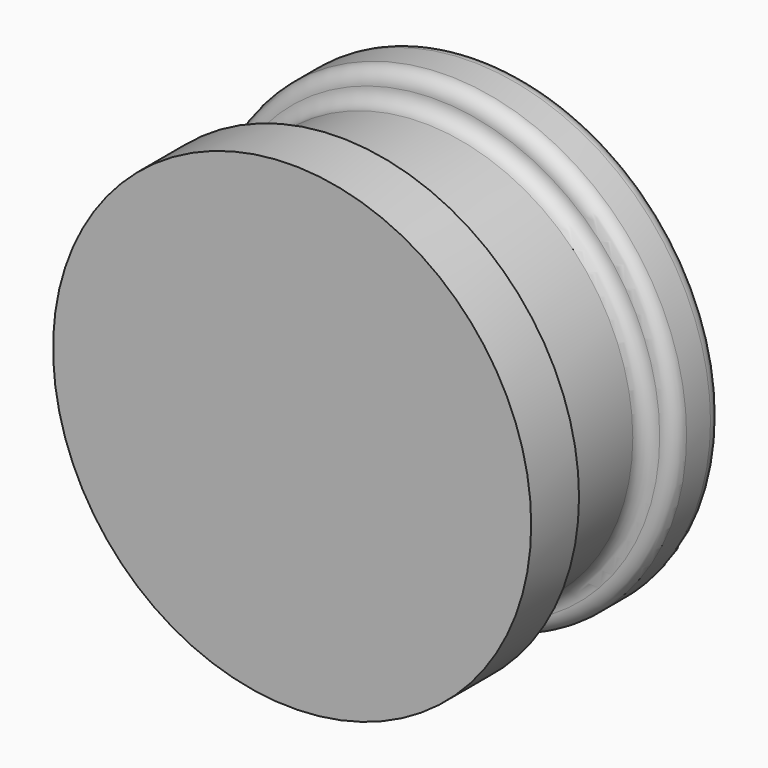
from build123d import *

# Parameters (mm, degrees)
F0_R      = 25.4
F1_DEPTH  = 6.35
F2_R      = 22.225
F3_DEPTH  = 12.7
F4_R      = 25.4
F4_R_2    = 22.225
F5_DEPTH  = 6.35
F7_D      = 3.175
F7_DEPTH  = 3.175
F7_TIP    = 0.9538662327
F8_D      = 12.7
F9_R      = 1.58749
F10_DEPTH = 6.35


# Not quite as in the source:
# - a fillet or chamfer is up to 0.001 mm smaller than in the source, because OpenCascade refuses the exact size


with BuildPart() as f1:
    # F0 (on Front) → F1 (new body)
    with BuildSketch(Plane.XZ):
        with Locations((0, -3.2290907108)):
            Circle(F0_R)
    extrude(amount=F1_DEPTH)

    # F2 (on face) → F3 (join)
    with BuildSketch(Plane.XZ.offset(6.35)):
        with Locations((0, -3.2290907108)):
            Circle(F2_R)
    extrude(amount=F3_DEPTH)

    # F4 (on face) → F5 (join)
    with BuildSketch(Plane.XZ.offset(19.05)):
        with Locations((0, -3.2290907108)):
            Circle(F4_R)
        with Locations((0, -3.2290907108)):
            Circle(F4_R_2, mode=Mode.SUBTRACT)
        with Locations((0, -3.2290907108)):
            Circle(F4_R_2)
    extrude(amount=F5_DEPTH)

    # F7
    with Locations(Plane.XZ.offset(25.4)):
        with Locations((19.05, -3.2290907108), (0, -22.2790907108), (-19.05, -3.2290907108), (0, 15.8209092892)):
            Hole(F7_D / 2, depth=F7_DEPTH)
            with Locations((0, 0, -(F7_DEPTH + F7_TIP / 2))):  # 118° drill point
                Cone(0, F7_D / 2, F7_TIP, mode=Mode.SUBTRACT)

    # F8 (through all)
    with Locations(Plane(origin=(0, 0, 0), x_dir=(1, 0, 0), z_dir=(0, 1, 0))):
        with Locations((0, 3.2290907108)):
            Hole(F8_D / 2)

    # F9 (radius 1.5875 in the source; OpenCascade refuses exactly that, so slightly less here)
    f9_edges = [f1.edges().sort_by_distance(p)[0] for p in [
        (-25.4, -6.35, -3.229091),
        (-25.4, 0, -3.229091),
        (-22.225, -6.35, -3.229091),
        (-25.4, -25.4, -3.229091),
        (-25.4, -19.05, -3.229091),
        (-22.225, -19.05, -3.229091),
    ]]
    fillet(f9_edges, radius=F9_R)

    # F4 (on face) → F10 (join)
    with BuildSketch(Plane.XZ.offset(19.05)):
        with Locations((0, -3.2290907108)):
            Circle(F4_R)
    extrude(amount=F10_DEPTH)


solid = f1.part
